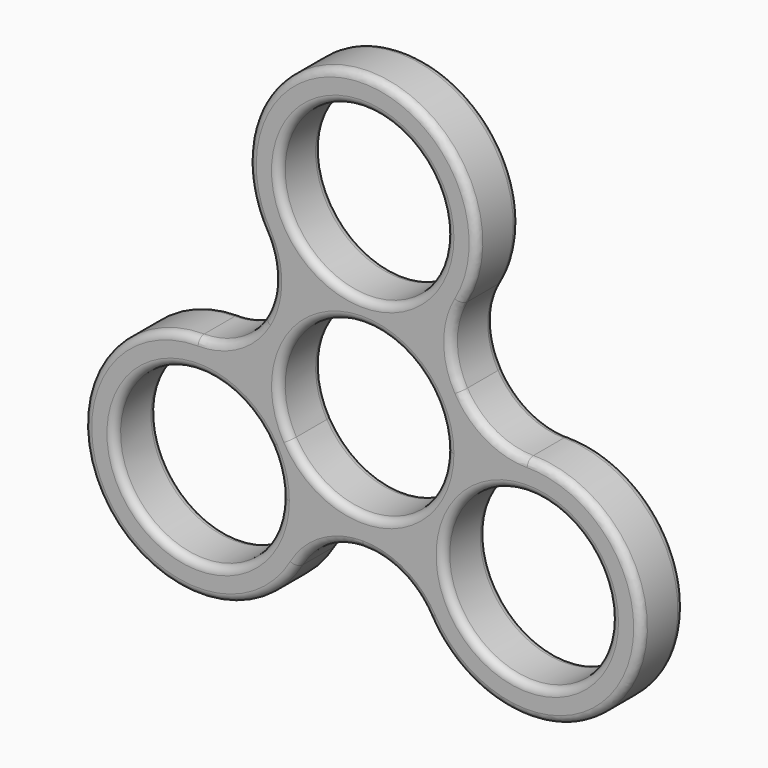
from build123d import *

# Parameters (mm, degrees)
F0_R     = 11
F1_DEPTH = 7
F2_R     = 9.999
F3_R     = 1


# Not quite as in the source:
# - a fillet or chamfer is up to 0.001 mm smaller than in the source, because OpenCascade refuses the exact size


with BuildPart() as f1:
    # F0 (on Front) → F1 (new body)
    with BuildSketch(Plane.XZ):
        with BuildLine():
            ThreePointArc((8.2915619759, 12.5), (0, 40), (-8.2915619759, 12.5))
            ThreePointArc((-8.2915619759, 12.5), (-12.9903810568, 7.5), (-14.9710985352, 0.9307033082))
            ThreePointArc((-14.9710985352, 0.9307033082), (-34.6410161514, -20), (-6.6795365594, -13.4307033082))
            ThreePointArc((-6.6795365594, -13.4307033082), (0, -15), (6.6795365594, -13.4307033082))
            ThreePointArc((6.6795365594, -13.4307033082), (34.6410161514, -20), (14.9710985352, 0.9307033082))
            ThreePointArc((14.9710985352, 0.9307033082), (12.9903810568, 7.5), (8.2915619759, 12.5))
        make_face()
        with BuildLine():
            ThreePointArc((-10.6506350946, -12.5), (-32.2758191838, -15.3470094961), (-12.124355653, -7))
            ThreePointArc((-12.124355653, -7), (-11.0254510054, -9.6529905039), (-10.6506350946, -12.5))
        make_face(mode=Mode.SUBTRACT)
        with BuildLine():
            ThreePointArc((-9.5262794416, -5.5), (-2.8470094961, 10.6251840892), (11, 0))
            ThreePointArc((11, 0), (2.8470094961, -10.6251840892), (-9.5262794416, -5.5))
        make_face(mode=Mode.SUBTRACT)
        with Locations((21.6506350946, -12.5)):
            Circle(F0_R, mode=Mode.SUBTRACT)
        with Locations((0, 25)):
            Circle(F0_R, mode=Mode.SUBTRACT)
    extrude(amount=F1_DEPTH)

    # F2 (radius 10 in the source; OpenCascade refuses exactly that, so slightly less here)
    f2_edges = [f1.edges().sort_by_distance(p)[0] for p in [
        (-6.679537, -3.5, -13.430703),
        (6.679537, -3.5, -13.430703),
        (14.971099, -3.5, 0.930703),
        (8.291562, -3.5, 12.5),
        (-8.291562, -3.5, 12.5),
        (-14.971099, -3.5, 0.930703),
    ]]
    fillet(f2_edges, radius=F2_R)

    # F3
    f3_edges = [f1.edges().sort_by_distance(p)[0] for p in [
        (-31.176915, 0, -18),
        (-11, 0, 0),
        (-11.65048, 0, 12.5),
        (-34.641016, 0, -20),
        (-11, 0, 25),
        (-11, -7, 25),
        (-11, -7, 0),
        (-31.176915, -7, -18),
        (10.650635, 0, -12.5),
        (10.650635, -7, -12.5),
        (-34.641016, -7, -20),
        (-11.65048, -7, 12.5),
    ]]
    fillet(f3_edges, radius=F3_R)


solid = f1.part
